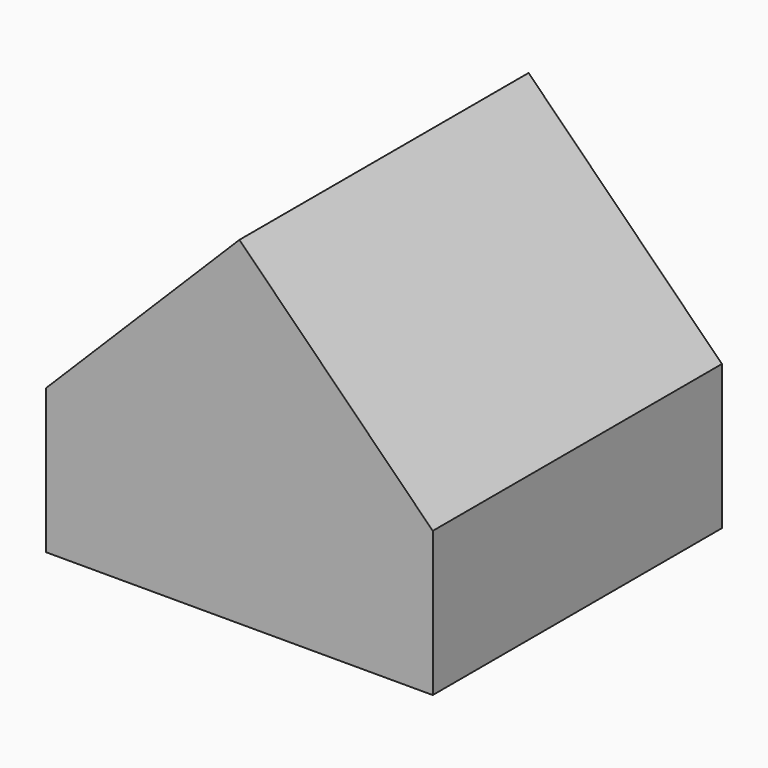
from build123d import *

# Parameters (mm, degrees)
F0_W        = 53.4896697645
F0_H        = 50
F1_DEPTH    = 50
F2_T1_DEPTH = 204.300979278


# Not quite as in the source:
# - a fillet or chamfer that OpenCascade refuses, or shapes differently, is made with other operations: its cross-section is extruded or revolved along the edge and cut away or added


with BuildPart() as f1:
    # F0 (on Front) → F1 (new body)
    with BuildSketch(Plane.XZ):
        with Locations((26.7448348823, 25)):
            Rectangle(F0_W, F0_H)
    extrude(amount=F1_DEPTH)

    # F2: chamfer of 30 on 2 edges, made by hand

    # F2_s2 → F2_t1 (cut)
    with BuildSketch(Plane.XZ.offset(-77.150489639)):
        Polygon((53.4896697645, 20), (23.4896697645, 50), (53.4896697645, 50), align=None)
        Polygon((0, 20), (30, 50), (0, 50), align=None)
    extrude(amount=F2_T1_DEPTH, mode=Mode.SUBTRACT)


solid = f1.part
